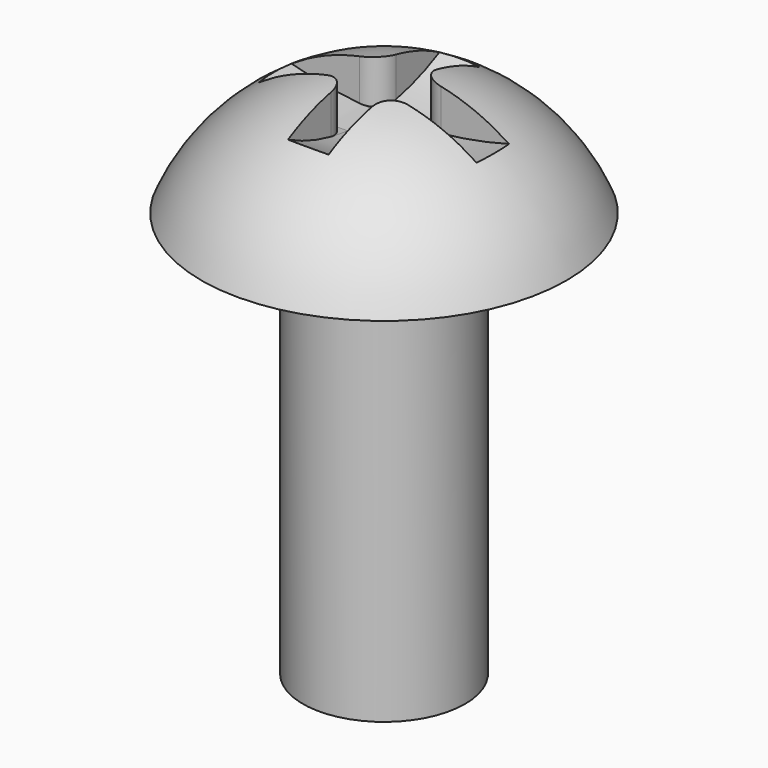
from build123d import *

# Parameters (mm, degrees)
F0_R         = 2
F1_DEPTH     = 10
F5_DEPTH     = 0.5
F7_DEPTH     = 0.5
F8_T4_DEPTH  = 3.6233825309
F8_S5_R      = 10
F8_T6_DEPTH  = 3
F8_S7_R      = 5
F8_T8_DEPTH  = 3
F8_T12_DEPTH = 3.6233825309
F8_S13_R     = 10
F8_T14_DEPTH = 3
F8_S15_R     = 5
F8_T16_DEPTH = 3
F8_T20_DEPTH = 3.6233825309
F8_S21_R     = 10
F8_T22_DEPTH = 3
F8_S23_R     = 5
F8_T24_DEPTH = 3
F8_T28_DEPTH = 3.6233825309
F8_S29_R     = 10
F8_T30_DEPTH = 3
F8_S31_R     = 5
F8_T32_DEPTH = 3


# Not quite as in the source:
# - a fillet or chamfer that OpenCascade refuses, or shapes differently, is made with other operations: its cross-section is extruded or revolved along the edge and cut away or added


with BuildPart() as f1:
    # F0 (on Top) → F1 (new body)
    with BuildSketch(Plane.XY):
        Circle(F0_R)
    extrude(amount=F1_DEPTH)

    # F2 (on Front) → F3 (revolve)
    with BuildSketch(Plane.XZ):
        with BuildLine():
            Line((0, 10), (4.5, 10))
            ThreePointArc((4.5, 10), (2.7041634566, 12.1812451849), (0, 13))
            Line((0, 13), (0, 10))
        make_face()
    revolve(axis=Axis((0, 0, 12.25), (0, 0, -1)))

    # F4 (on Front) → F5 (cut, symmetric)
    with BuildSketch(Plane.XZ):
        with BuildLine():
            ThreePointArc((-2.7226391671, 12.177773856), (0, 11.8), (2.7226391671, 12.177773856))
            ThreePointArc((2.7226391671, 12.177773856), (0, 13), (-2.7226391671, 12.177773856))
        make_face()
    extrude(amount=F5_DEPTH, both=True, mode=Mode.SUBTRACT)

    # F6 (on Right) → F7 (cut, symmetric)
    with BuildSketch(Plane.YZ):
        with BuildLine():
            ThreePointArc((-2.3644931313, 12.3944157899), (0, 11.8), (2.3644931313, 12.3944157899))
            ThreePointArc((2.3644931313, 12.3944157899), (0, 13), (-2.3644931313, 12.3944157899))
        make_face()
    extrude(amount=F7_DEPTH, both=True, mode=Mode.SUBTRACT)

    # F8: fillet of radius 0.5 on 4 edges, made by hand


with BuildPart() as f8_tool2:
    # F8_s3 → F8_t4 (new body)
    with BuildSketch(Plane.XY.offset(10.5750628145)):
        with BuildLine():
            ThreePointArc((1, -0.5), (0.6464466094, -0.6464466094), (0.5, -1))
            Line((0.5, -1), (0.5, -0.5))
            Line((0.5, -0.5), (1, -0.5))
        make_face()
    extrude(amount=F8_T4_DEPTH)

    # F8_s5 → F8_t6 (intersect, symmetric)
    with BuildSketch(Plane.XZ.offset(0.8)):
        with Locations((0, 21.8)):
            Circle(F8_S5_R)
    extrude(amount=F8_T6_DEPTH, both=True, mode=Mode.INTERSECT)

    # F8_s7 → F8_t8 (intersect, symmetric)
    with BuildSketch(Plane.YZ.offset(0.8)):
        with Locations((0, 16.8)):
            Circle(F8_S7_R)
    extrude(amount=F8_T8_DEPTH, both=True, mode=Mode.INTERSECT)


with BuildPart() as f1_1:
    add(f1.part)

    # F8_t1: cut F8_tool2
    add(f8_tool2.part, mode=Mode.SUBTRACT)


with BuildPart() as f8_tool10:
    # F8_s11 → F8_t12 (new body)
    with BuildSketch(Plane.XY.offset(10.5750628145)):
        with BuildLine():
            ThreePointArc((-1, -0.5), (-0.6464466094, -0.6464466094), (-0.5, -1))
            Line((-0.5, -1), (-0.5, -0.5))
            Line((-0.5, -0.5), (-1, -0.5))
        make_face()
    extrude(amount=F8_T12_DEPTH)

    # F8_s13 → F8_t14 (intersect, symmetric)
    with BuildSketch(Plane.XZ.offset(0.8)):
        with Locations((0, 21.8)):
            Circle(F8_S13_R)
    extrude(amount=F8_T14_DEPTH, both=True, mode=Mode.INTERSECT)

    # F8_s15 → F8_t16 (intersect, symmetric)
    with BuildSketch(Plane.YZ.offset(-0.8)):
        with Locations((0, 16.8)):
            Circle(F8_S15_R)
    extrude(amount=F8_T16_DEPTH, both=True, mode=Mode.INTERSECT)


with BuildPart() as f1_2:
    add(f1_1.part)

    # F8_t9: cut F8_tool10
    add(f8_tool10.part, mode=Mode.SUBTRACT)


with BuildPart() as f8_tool18:
    # F8_s19 → F8_t20 (new body)
    with BuildSketch(Plane.XY.offset(10.5750628145)):
        with BuildLine():
            ThreePointArc((-1, 0.5), (-0.6464466094, 0.6464466094), (-0.5, 1))
            Line((-0.5, 1), (-0.5, 0.5))
            Line((-0.5, 0.5), (-1, 0.5))
        make_face()
    extrude(amount=F8_T20_DEPTH)

    # F8_s21 → F8_t22 (intersect, symmetric)
    with BuildSketch(Plane.XZ.offset(-0.7)):
        with Locations((0, 21.8)):
            Circle(F8_S21_R)
    extrude(amount=F8_T22_DEPTH, both=True, mode=Mode.INTERSECT)

    # F8_s23 → F8_t24 (intersect, symmetric)
    with BuildSketch(Plane.YZ.offset(-0.8)):
        with Locations((0, 16.8)):
            Circle(F8_S23_R)
    extrude(amount=F8_T24_DEPTH, both=True, mode=Mode.INTERSECT)


with BuildPart() as f1_3:
    add(f1_2.part)

    # F8_t17: cut F8_tool18
    add(f8_tool18.part, mode=Mode.SUBTRACT)


with BuildPart() as f8_tool26:
    # F8_s27 → F8_t28 (new body)
    with BuildSketch(Plane.XY.offset(10.5750628145)):
        with BuildLine():
            ThreePointArc((1, 0.5), (0.6464466094, 0.6464466094), (0.5, 1))
            Line((0.5, 1), (0.5, 0.5))
            Line((0.5, 0.5), (1, 0.5))
        make_face()
    extrude(amount=F8_T28_DEPTH)

    # F8_s29 → F8_t30 (intersect, symmetric)
    with BuildSketch(Plane.XZ.offset(-0.7)):
        with Locations((0, 21.8)):
            Circle(F8_S29_R)
    extrude(amount=F8_T30_DEPTH, both=True, mode=Mode.INTERSECT)

    # F8_s31 → F8_t32 (intersect, symmetric)
    with BuildSketch(Plane.YZ.offset(0.8)):
        with Locations((0, 16.8)):
            Circle(F8_S31_R)
    extrude(amount=F8_T32_DEPTH, both=True, mode=Mode.INTERSECT)


with BuildPart() as f1_4:
    add(f1_3.part)

    # F8_t25: cut F8_tool26
    add(f8_tool26.part, mode=Mode.SUBTRACT)


solid = f1_4.part
